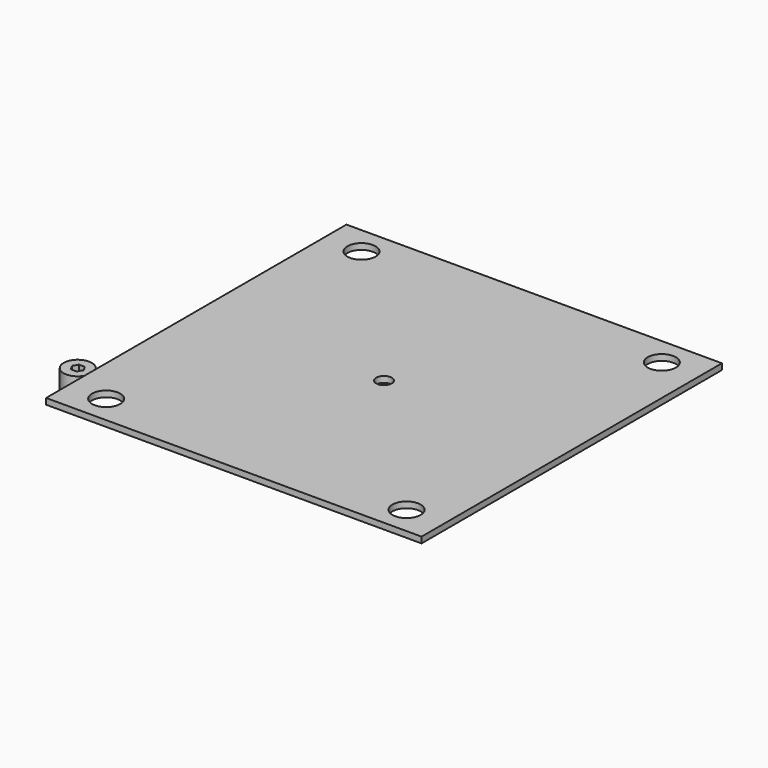
from build123d import *

# Parameters (mm, degrees)
F0_W     = 200
F0_H     = 200
F0_R     = 7.5
F0_R_2   = 4.15
F1_DEPTH = 3.2
F2_R     = 7.5
F3_DEPTH = 12


with BuildPart() as f1:
    # F0 (on Top) → F1 (new body)
    with BuildSketch(Plane.XY):
        with Locations((0, 37.4703630805)):
            Rectangle(F0_W, F0_H)
        with Locations((-80, -47.5296369195)):
            Circle(F0_R, mode=Mode.SUBTRACT)
        with Locations((80, -47.5296369195)):
            Circle(F0_R, mode=Mode.SUBTRACT)
        with Locations((0, 37.4703630805)):
            Circle(F0_R_2, mode=Mode.SUBTRACT)
        with Locations((-80, 122.4703630805)):
            Circle(F0_R, mode=Mode.SUBTRACT)
        with Locations((80, 122.4703630805)):
            Circle(F0_R, mode=Mode.SUBTRACT)
    extrude(amount=-F1_DEPTH)


with BuildPart() as f3:
    # F2 (on face) → F3 (new body)
    with BuildSketch(Plane(origin=(0, 0, -3.2), x_dir=(1, 0, 0), z_dir=(0, 0, -1))):
        with Locations((-110.3689859124, 28.4748198305)):
            Circle(F2_R)
        Polygon((-113.4869859124, 28.4748198305), (-111.9279859124, 31.1750870395), (-108.8099859124, 31.1750870395), (-107.2509859124, 28.4748198305), (-108.8099859124, 25.7745526215), (-111.9279859124, 25.7745526215), align=None, mode=Mode.SUBTRACT)
    extrude(amount=F3_DEPTH)


solid = Compound([f1.part, f3.part])
